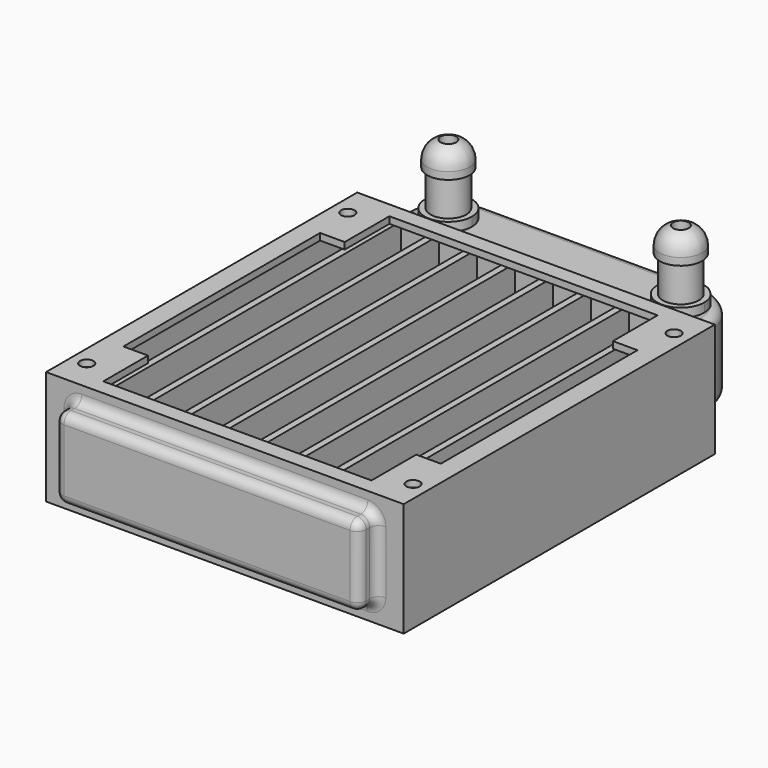
from build123d import *

# Parameters (mm, degrees)
F0_R      = 1.5
F1_DEPTH  = 1.5
F2_W      = 80
F2_H      = 87
F2_W_2    = 1.5
F2_H_2    = 80
F2_H_3    = 2
F3_DEPTH  = 22.5
F4_START  = 24
F4_DEPTH  = 1.5
F6_START  = -87
F5_W      = 68
F5_H      = 18
F6_DEPTH  = 5
F7_DEPTH  = 16
F8_R      = 10
F9_R      = 2
F10_R     = 4.75
F10_R_2   = 4
F11_DEPTH = 2
F10_R_3   = 1.75
F12_DEPTH = 10
F13_START = 10
F13_DEPTH = 5.5


# Not quite as in the source:
# - a fillet or chamfer that OpenCascade refuses, or shapes differently, is made with other operations: its cross-section is extruded or revolved along the edge and cut away or added


with BuildPart() as f1:
    # F0 (on Top) → F1 (new body)
    with BuildSketch(Plane.XY):
        Polygon((30, 43.5), (-40, 43.5), (-40, -43.5), (40, -43.5), (40, 27.5), (40, 43.5), align=None)
        with Locations((-36.5, -36.5)):
            Circle(F0_R, mode=Mode.SUBTRACT)
        with Locations((36.5, -36.5)):
            Circle(F0_R, mode=Mode.SUBTRACT)
        with Locations((-36.5, 36.5)):
            Circle(F0_R, mode=Mode.SUBTRACT)
        Polygon((30, 27.5), (35.5, 27.5), (35.5, -27.5), (30, -27.5), (30, -40), (-30, -40), (-30, -27.5), (-35.5, -27.5), (-35.5, 27.5), (-30, 27.5), (-30, 40), (30, 40), align=None, mode=Mode.SUBTRACT)
        with Locations((36.5, 36.5)):
            Circle(F0_R, mode=Mode.SUBTRACT)
    extrude(amount=F1_DEPTH)

    # F2 (on face) → F3 (join)
    with BuildSketch(Plane.XY.offset(1.5)):
        Rectangle(F2_W, F2_H)
        Polygon((-38.5, -42), (-38.5, 42), (-30.5, 42), (-29, 42), (-22, 42), (-20.5, 42), (-13.5, 42), (-12, 42), (-5, 42), (-3.5, 42), (3.5, 42), (5, 42), (12, 42), (13.5, 42), (20.5, 42), (22, 42), (29, 42), (30.5, 42), (38.5, 42), (38.5, -42), (30.5, -42), (29, -42), (22, -42), (20.5, -42), (13.5, -42), (12, -42), (5, -42), (3.5, -42), (-3.5, -42), (-5, -42), (-12, -42), (-13.5, -42), (-20.5, -42), (-22, -42), (-29, -42), (-30.5, -42), align=None, mode=Mode.SUBTRACT)
        Polygon((-30, 27.5), (-30.5, 27.5), (-30.5, -27.5), (-30, -27.5), (-30, -40), (-29, -40), (-29, 40), (-30, 40), align=None)
        Polygon((-29, 42), (-30.5, 42), (-30.5, 27.5), (-30, 27.5), (-30, 40), (-29, 40), align=None)
        with Locations((-21.25, 0)):
            Rectangle(F2_W_2, F2_H_2)
        with Locations((-12.75, 0)):
            Rectangle(F2_W_2, F2_H_2)
        with Locations((-4.25, 0)):
            Rectangle(F2_W_2, F2_H_2)
        with Locations((4.25, 0)):
            Rectangle(F2_W_2, F2_H_2)
        with Locations((12.75, 0)):
            Rectangle(F2_W_2, F2_H_2)
        with Locations((21.25, 0)):
            Rectangle(F2_W_2, F2_H_2)
        Polygon((30, 40), (29, 40), (29, -40), (30, -40), (30, -27.5), (30.5, -27.5), (30.5, 27.5), (30, 27.5), align=None)
        Polygon((29, -40), (29, -42), (30.5, -42), (30.5, -27.5), (30, -27.5), (30, -40), align=None)
        Polygon((30.5, 42), (29, 42), (29, 40), (30, 40), (30, 27.5), (30.5, 27.5), align=None)
        Polygon((-30.5, -27.5), (-30.5, -42), (-29, -42), (-29, -40), (-30, -40), (-30, -27.5), align=None)
        with Locations((21.25, -41)):
            Rectangle(F2_W_2, F2_H_3)
        with Locations((12.75, -41)):
            Rectangle(F2_W_2, F2_H_3)
        with Locations((-4.25, -41)):
            Rectangle(F2_W_2, F2_H_3)
        with Locations((4.25, -41)):
            Rectangle(F2_W_2, F2_H_3)
        with Locations((-12.75, -41)):
            Rectangle(F2_W_2, F2_H_3)
        with Locations((-21.25, -41)):
            Rectangle(F2_W_2, F2_H_3)
        with Locations((21.25, 41)):
            Rectangle(F2_W_2, F2_H_3)
        with Locations((12.75, 41)):
            Rectangle(F2_W_2, F2_H_3)
        with Locations((4.25, 41)):
            Rectangle(F2_W_2, F2_H_3)
        with Locations((-4.25, 41)):
            Rectangle(F2_W_2, F2_H_3)
        with Locations((-12.75, 41)):
            Rectangle(F2_W_2, F2_H_3)
        with Locations((-21.25, 41)):
            Rectangle(F2_W_2, F2_H_3)
    extrude(amount=F3_DEPTH)

    # F0 (on Top) → F4 (join)
    with BuildSketch(Plane.XY.offset(F4_START)):
        Polygon((30, 43.5), (-40, 43.5), (-40, -43.5), (40, -43.5), (40, 27.5), (40, 43.5), align=None)
        with Locations((-36.5, -36.5)):
            Circle(F0_R, mode=Mode.SUBTRACT)
        with Locations((36.5, -36.5)):
            Circle(F0_R, mode=Mode.SUBTRACT)
        with Locations((-36.5, 36.5)):
            Circle(F0_R, mode=Mode.SUBTRACT)
        Polygon((30, 27.5), (35.5, 27.5), (35.5, -27.5), (30, -27.5), (30, -40), (-30, -40), (-30, -27.5), (-35.5, -27.5), (-35.5, 27.5), (-30, 27.5), (-30, 40), (30, 40), align=None, mode=Mode.SUBTRACT)
        with Locations((36.5, 36.5)):
            Circle(F0_R, mode=Mode.SUBTRACT)
    extrude(amount=F4_DEPTH)

    # F5 (on face) → F6 (join)
    with BuildSketch(Plane(origin=(0, 43.5, 0), x_dir=(-1, 0, 0), z_dir=(0, 1, 0)).offset(F6_START)):
        with Locations((0, 12.75)):
            Rectangle(F5_W, F5_H)
    extrude(amount=-F6_DEPTH)

    # F5 (on face) → F7 (join)
    with BuildSketch(Plane(origin=(0, 43.5, 0), x_dir=(-1, 0, 0), z_dir=(0, 1, 0))):
        with Locations((0, 12.75)):
            Rectangle(F5_W, F5_H)
    extrude(amount=F7_DEPTH)

    # F8
    f8_edges = [f1.edges().sort_by_distance(p)[0] for p in [
        (34, 59.5, 12.75),
        (-34, 59.5, 12.75),
    ]]
    fillet(f8_edges, radius=F8_R)

    # F9
    f9_edges = [f1.edges().sort_by_distance(p)[0] for p in [
        (34, 46.5, 3.75),
        (31.071068, 56.571068, 3.75),
        (0, 43.5, 3.75),
        (0, 59.5, 3.75),
        (-34, 46.5, 3.75),
        (-31.071068, 56.571068, 3.75),
        (-34, 46.5, 21.75),
        (-31.071068, 56.571068, 21.75),
        (0, 43.5, 21.75),
        (0, 59.5, 21.75),
        (34, 46.5, 21.75),
        (31.071068, 56.571068, 21.75),
        (0, -48.5, 21.75),
        (34, -48.5, 12.75),
        (0, -48.5, 3.75),
        (-34, -48.5, 12.75),
        (0, -43.5, 21.75),
        (34, -43.5, 12.75),
        (0, -43.5, 3.75),
        (-34, -43.5, 12.75),
        (-34, -46, 21.75),
        (-34, -46, 3.75),
        (34, -46, 3.75),
        (34, -46, 21.75),
        (-34, 43.5, 12.75),
        (34, 43.5, 12.75),
    ]]
    fillet(f9_edges, radius=F9_R)

    # F10 (on face) → F11 (join)
    with BuildSketch(Plane.XY.offset(21.75)):
        with BuildLine():
            ThreePointArc((-30.6249429729, 53.9844320271), (-27.2809272798, 46.4086617374), (-20.75, 51.5))
            ThreePointArc((-20.75, 51.5), (-23.3056325549, 56.0058721765), (-28.4844320271, 56.1249429729))
            ThreePointArc((-28.4844320271, 56.1249429729), (-29.6568542495, 55.1568542495), (-30.6249429729, 53.9844320271))
        make_face()
        with Locations((-26, 51.5)):
            Circle(F10_R, mode=Mode.SUBTRACT)
        with Locations((-26, 51.5)):
            Circle(F10_R)
        with Locations((-26, 51.5)):
            Circle(F10_R_2, mode=Mode.SUBTRACT)
        with BuildLine():
            ThreePointArc((30.6249429729, 53.9844320271), (29.6568542495, 55.1568542495), (28.4844320271, 56.1249429729))
            ThreePointArc((28.4844320271, 56.1249429729), (21.4941278235, 48.8056325549), (31.25, 51.5))
            ThreePointArc((31.25, 51.5), (31.0913382626, 52.7809272798), (30.6249429729, 53.9844320271))
        make_face()
        with Locations((26, 51.5)):
            Circle(F10_R, mode=Mode.SUBTRACT)
        with Locations((26, 51.5)):
            Circle(F10_R)
        with Locations((26, 51.5)):
            Circle(F10_R_2, mode=Mode.SUBTRACT)
    extrude(amount=F11_DEPTH)

    # F10 (on face) → F12 (join)
    with BuildSketch(Plane.XY.offset(21.75)):
        with Locations((-26, 51.5)):
            Circle(F10_R_2)
        with Locations((-26, 51.5)):
            Circle(F10_R_3, mode=Mode.SUBTRACT)
        with Locations((26, 51.5)):
            Circle(F10_R_2)
        with Locations((26, 51.5)):
            Circle(F10_R_3, mode=Mode.SUBTRACT)
    extrude(amount=F12_DEPTH)

    # F10 (on face) → F13 (join)
    with BuildSketch(Plane.XY.offset(21.75).offset(F13_START)):
        with Locations((-26, 51.5)):
            Circle(F10_R)
        with Locations((-26, 51.5)):
            Circle(F10_R_2, mode=Mode.SUBTRACT)
        with Locations((26, 51.5)):
            Circle(F10_R)
        with Locations((26, 51.5)):
            Circle(F10_R_2, mode=Mode.SUBTRACT)
        with Locations((-26, 51.5)):
            Circle(F10_R_2)
        with Locations((-26, 51.5)):
            Circle(F10_R_3, mode=Mode.SUBTRACT)
        with Locations((26, 51.5)):
            Circle(F10_R_2)
        with Locations((26, 51.5)):
            Circle(F10_R_3, mode=Mode.SUBTRACT)
    extrude(amount=F13_DEPTH)

    # F14: fillet of radius 4 on 2 edges, made by hand

    # F14_s1 → F14_t2 (revolve, cut)
    with BuildSketch(Plane.XZ.offset(-51.5)):
        with BuildLine():
            ThreePointArc((-21.25, 33.3770166538), (-22.0877223398, 35.8265063966), (-24.25, 37.25))
            Line((-24.25, 37.25), (-21.25, 37.25))
            Line((-21.25, 37.25), (-21.25, 33.3770166538))
        make_face()
    revolve(axis=Axis((-26, 51.5, 37.25), (0, 0, 1)), mode=Mode.SUBTRACT)

    # F14_s3 → F14_t4 (revolve, cut)
    with BuildSketch(Plane.XZ.offset(-51.5)):
        with BuildLine():
            ThreePointArc((30.75, 33.3770166538), (29.9122776602, 35.8265063966), (27.75, 37.25))
            Line((27.75, 37.25), (30.75, 37.25))
            Line((30.75, 37.25), (30.75, 33.3770166538))
        make_face()
    revolve(axis=Axis((26, 51.5, 37.25), (0, 0, 1)), mode=Mode.SUBTRACT)


solid = f1.part
